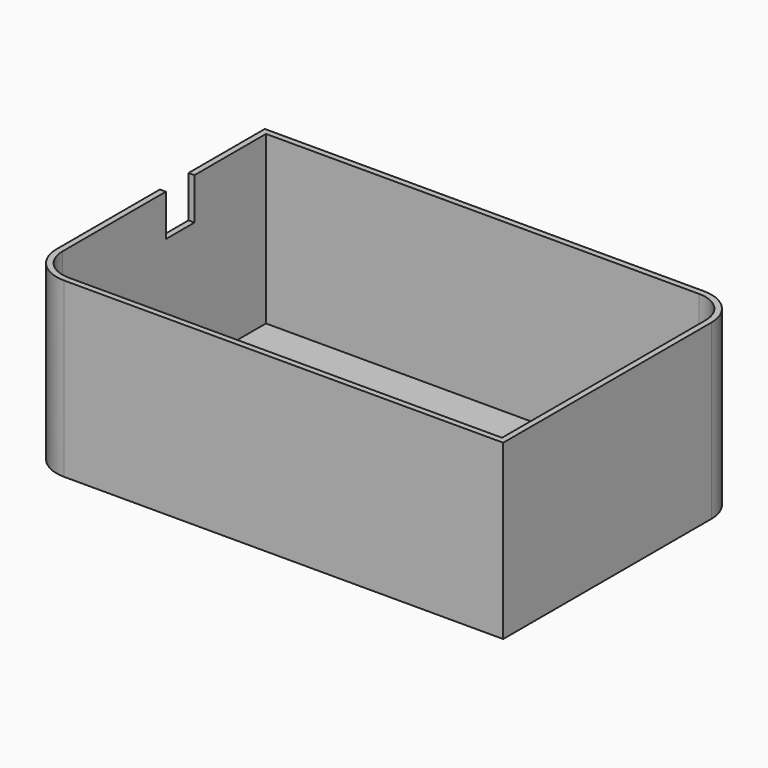
from build123d import *

# Parameters (mm, degrees)
F1_DEPTH = 29
F3_DEPTH = 28
F4_W     = 6
F4_H     = 7
F5_DEPTH = 44.45


# Not quite as in the source:
# - a feature names something its author has since deleted; it is built from what else it names


with BuildPart() as f1:
    # F0 (on Top) → F1 (new body)
    with BuildSketch(Plane.XY):
        with BuildLine():
            Line((-33.65, -25), (40, -25))
            Line((40, -25), (40, 18.65))
            ThreePointArc((40, 18.65), (38.1401280605, 23.1401280605), (33.65, 25))
            Line((33.65, 25), (-40, 25))
            Line((-40, 25), (-40, -18.65))
            ThreePointArc((-40, -18.65), (-38.1401280605, -23.1401280605), (-33.65, -25))
        make_face()
    extrude(amount=F1_DEPTH)

    # F2 (on face) → F3 (cut)
    with BuildSketch(Plane.XY.offset(29)):
        with BuildLine():
            Line((33.666, 24), (-39, 24))
            Line((-39, 24), (-39, -18.666))
            ThreePointArc((-39, -18.666), (-37.4377075708, -22.4377075708), (-33.666, -24))
            Line((-33.666, -24), (39, -24))
            Line((39, -24), (39, 18.666))
            ThreePointArc((39, 18.666), (37.4377075708, 22.4377075708), (33.666, 24))
        make_face()
    extrude(amount=-F3_DEPTH, mode=Mode.SUBTRACT)

    # F4 (on face) → F5 (cut)
    with BuildSketch(Plane.YZ.offset(-39)):
        with Locations((6, 25.5)):
            Rectangle(F4_W, F4_H)
    extrude(amount=-F5_DEPTH, mode=Mode.SUBTRACT)


solid = f1.part
